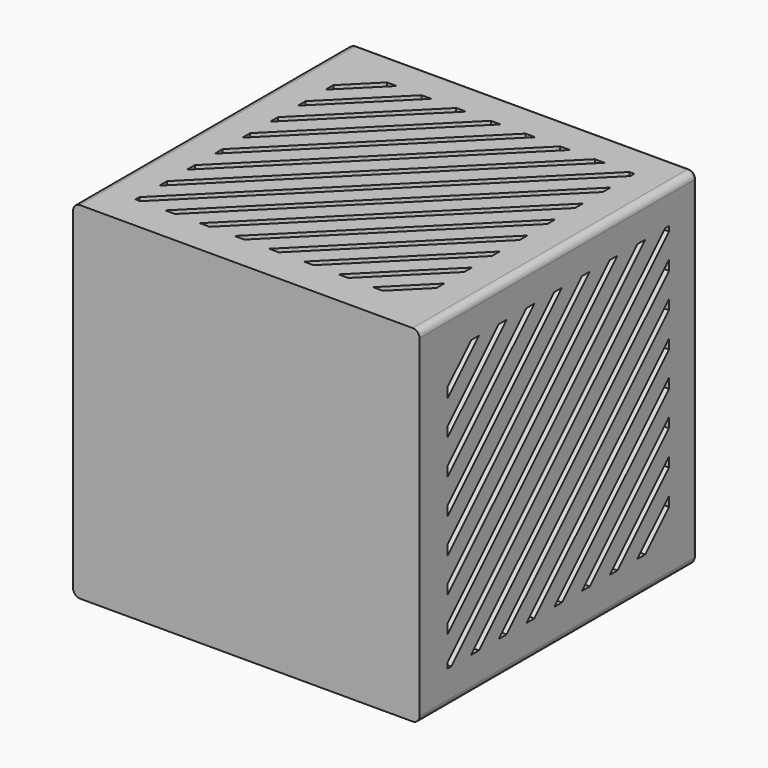
from build123d import *

# Parameters (mm, degrees)
F0_W         = 100
F0_H         = 100
F1_DEPTH     = 100
F3_T         = -2.5
F4_DEPTH     = 102
F6_DEPTH     = 108.7
F7_R         = 1
F8_T1_DEPTH  = 105
F8_T4_ANGLE  = 90
F9_T1_DEPTH  = 105
F9_T4_ANGLE  = 90
F10_T1_DEPTH = 105
F10_T4_ANGLE = 90
F11_T1_DEPTH = 105
F11_T4_ANGLE = 90


# Not quite as in the source:
# - a fillet or chamfer that OpenCascade refuses, or shapes differently, is made with other operations: its cross-section is extruded or revolved along the edge and cut away or added


with BuildPart() as f1:
    # F0 (on Top) → F1 (new body)
    with BuildSketch(Plane.XY):
        Rectangle(F0_W, F0_H)
    extrude(amount=F1_DEPTH)

    # F3
    f3_openings = [f1.faces().sort_by_distance(p)[0] for p in [
        (0, 50, 50),
    ]]
    offset(amount=F3_T, openings=f3_openings)

    # F2 (on face) → F4 (cut)
    with BuildSketch(Plane.XY.offset(100)):
        Polygon((-40, 28.5857864376), (-28.5857864376, 40), (-31.4142135624, 40), (-40, 31.4142135624), align=None)
        Polygon((-40, 18.5857864376), (-18.5857864376, 40), (-21.4142135624, 40), (-40, 21.4142135624), align=None)
        Polygon((-40, 8.5857864376), (-8.5857864376, 40), (-11.4142135624, 40), (-40, 11.4142135624), align=None)
        Polygon((-40, -1.4142135624), (1.4142135624, 40), (-1.4142135624, 40), (-40, 1.4142135624), align=None)
        Polygon((-40, -11.4142135624), (11.4142135624, 40), (8.5857864376, 40), (-40, -8.5857864376), align=None)
        Polygon((-40, -21.4142135624), (21.4142135624, 40), (18.5857864376, 40), (-40, -18.5857864376), align=None)
        Polygon((-40, -31.4142135624), (31.4142135624, 40), (28.5857864376, 40), (-40, -28.5857864376), align=None)
        Polygon((40, 38.5857864376), (40, 40), (38.5857864376, 40), (-40, -38.5857864376), (-40, -40), (-38.5857864376, -40), align=None)
        Polygon((40, 28.5857864376), (40, 31.4142135624), (-31.4142135624, -40), (-28.5857864376, -40), align=None)
        Polygon((40, 18.5857864376), (40, 21.4142135624), (-21.4142135624, -40), (-18.5857864376, -40), align=None)
        Polygon((40, 8.5857864376), (40, 11.4142135624), (-11.4142135624, -40), (-8.5857864376, -40), align=None)
        Polygon((40, -1.4142135624), (40, 1.4142135624), (-1.4142135624, -40), (1.4142135624, -40), align=None)
        Polygon((40, -11.4142135624), (40, -8.5857864376), (8.5857864376, -40), (11.4142135624, -40), align=None)
        Polygon((40, -21.4142135624), (40, -18.5857864376), (18.5857864376, -40), (21.4142135624, -40), align=None)
        Polygon((40, -31.4142135624), (40, -28.5857864376), (28.5857864376, -40), (31.4142135624, -40), align=None)
    extrude(amount=-F4_DEPTH, mode=Mode.SUBTRACT)

    # F5 (on face) → F6 (cut)
    with BuildSketch(Plane.YZ.offset(50)):
        Polygon((-40, 78.5857864376), (-28.5857864376, 90), (-31.4142135624, 90), (-40, 81.4142135624), align=None)
        Polygon((-40, 68.5857864376), (-18.5857864376, 90), (-21.4142135624, 90), (-40, 71.4142135624), align=None)
        Polygon((-40, 58.5857864376), (-8.5857864376, 90), (-11.4142135624, 90), (-40, 61.4142135624), align=None)
        Polygon((-40, 48.5857864376), (1.4142135624, 90), (-1.4142135624, 90), (-40, 51.4142135624), align=None)
        Polygon((-40, 38.5857864376), (11.4142135624, 90), (8.5857864376, 90), (-40, 41.4142135624), align=None)
        Polygon((-40, 28.5857864376), (21.4142135624, 90), (18.5857864376, 90), (-40, 31.4142135624), align=None)
        Polygon((-40, 18.5857864376), (31.4142135624, 90), (28.5857864376, 90), (-40, 21.4142135624), align=None)
        Polygon((40, 88.5857864376), (40, 90), (38.5857864376, 90), (-40, 11.4142135624), (-40, 10), (-38.5857864376, 10), align=None)
        Polygon((40, 78.5857864376), (40, 81.4142135624), (-31.4142135624, 10), (-28.5857864376, 10), align=None)
        Polygon((40, 68.5857864376), (40, 71.4142135624), (-21.4142135624, 10), (-18.5857864376, 10), align=None)
        Polygon((40, 58.5857864376), (40, 61.4142135624), (-11.4142135624, 10), (-8.5857864376, 10), align=None)
        Polygon((40, 48.5857864376), (40, 51.4142135624), (-1.4142135624, 10), (1.4142135624, 10), align=None)
        Polygon((11.4142135624, 10), (40, 38.5857864376), (40, 41.4142135624), (8.5857864376, 10), align=None)
        Polygon((21.4142135624, 10), (40, 28.5857864376), (40, 31.4142135624), (18.5857864376, 10), align=None)
        Polygon((31.4142135624, 10), (40, 18.5857864376), (40, 21.4142135624), (28.5857864376, 10), align=None)
    extrude(amount=-F6_DEPTH, mode=Mode.SUBTRACT)

    # F7
    f7_edges = [f1.edges().sort_by_distance(p)[0] for p in [
        (50, 50, 50),
        (0, 50, 100),
        (-50, 50, 50),
        (0, 50, 0),
        (47.5, 50, 50),
        (0, 50, 2.5),
        (-47.5, 50, 50),
        (0, 50, 97.5),
    ]]
    fillet(f7_edges, radius=F7_R)

    # F8: fillet of radius 2 on 1 edges, made by hand

    # F8_s2 → F8_t1 (cut)
    with BuildSketch(Plane.XZ.offset(-50)):
        with BuildLine():
            ThreePointArc((48, 0), (49.4142135624, 0.5857864376), (50, 2))
            Line((50, 2), (50, 0))
            Line((50, 0), (48, 0))
        make_face()
    extrude(amount=F8_T1_DEPTH, mode=Mode.SUBTRACT)

    # F8_s3 → F8_t4 (revolve, cut)
    with BuildSketch(Plane.XY.offset(2)):
        with BuildLine():
            ThreePointArc((49, 50), (49.7071067812, 49.7071067812), (50, 49))
            Line((50, 49), (50, 50))
            Line((50, 50), (49, 50))
        make_face()
    revolve(axis=Axis((48, 50, 2), (0, 1, 0)), revolution_arc=F8_T4_ANGLE, mode=Mode.SUBTRACT)

    # F9: fillet of radius 2 on 1 edges, made by hand

    # F9_s2 → F9_t1 (cut)
    with BuildSketch(Plane.XZ.offset(-50)):
        with BuildLine():
            ThreePointArc((-50, 2), (-49.4142135624, 0.5857864376), (-48, 0))
            Line((-48, 0), (-50, 0))
            Line((-50, 0), (-50, 2))
        make_face()
    extrude(amount=F9_T1_DEPTH, mode=Mode.SUBTRACT)

    # F9_s3 → F9_t4 (revolve, cut)
    with BuildSketch(Plane.YZ.offset(-48)):
        with BuildLine():
            ThreePointArc((50, 1), (49.7071067812, 0.2928932188), (49, 0))
            Line((49, 0), (50, 0))
            Line((50, 0), (50, 1))
        make_face()
    revolve(axis=Axis((-48, 50, 2), (0, 1, 0)), revolution_arc=F9_T4_ANGLE, mode=Mode.SUBTRACT)

    # F10: fillet of radius 2 on 1 edges, made by hand

    # F10_s2 → F10_t1 (cut)
    with BuildSketch(Plane.XZ.offset(-50)):
        with BuildLine():
            ThreePointArc((-50, 98), (-49.4142135624, 99.4142135624), (-48, 100))
            Line((-48, 100), (-50, 100))
            Line((-50, 100), (-50, 98))
        make_face()
    extrude(amount=F10_T1_DEPTH, mode=Mode.SUBTRACT)

    # F10_s3 → F10_t4 (revolve, cut)
    with BuildSketch(Plane.XY.offset(98)):
        with BuildLine():
            ThreePointArc((-49, 50), (-49.7071067812, 49.7071067812), (-50, 49))
            Line((-50, 49), (-50, 50))
            Line((-50, 50), (-49, 50))
        make_face()
    revolve(axis=Axis((-48, 50, 98), (0, 1, 0)), revolution_arc=F10_T4_ANGLE, mode=Mode.SUBTRACT)

    # F11: fillet of radius 2 on 1 edges, made by hand

    # F11_s2 → F11_t1 (cut)
    with BuildSketch(Plane.XZ.offset(-50)):
        with BuildLine():
            ThreePointArc((50, 98), (49.4142135624, 99.4142135624), (48, 100))
            Line((48, 100), (50, 100))
            Line((50, 100), (50, 98))
        make_face()
    extrude(amount=F11_T1_DEPTH, mode=Mode.SUBTRACT)

    # F11_s3 → F11_t4 (revolve, cut)
    with BuildSketch(Plane.YZ.offset(48)):
        with BuildLine():
            ThreePointArc((50, 99), (49.7071067812, 99.7071067812), (49, 100))
            Line((49, 100), (50, 100))
            Line((50, 100), (50, 99))
        make_face()
    revolve(axis=Axis((48, 50, 98), (0, 1, 0)), revolution_arc=F11_T4_ANGLE, mode=Mode.SUBTRACT)


solid = f1.part
